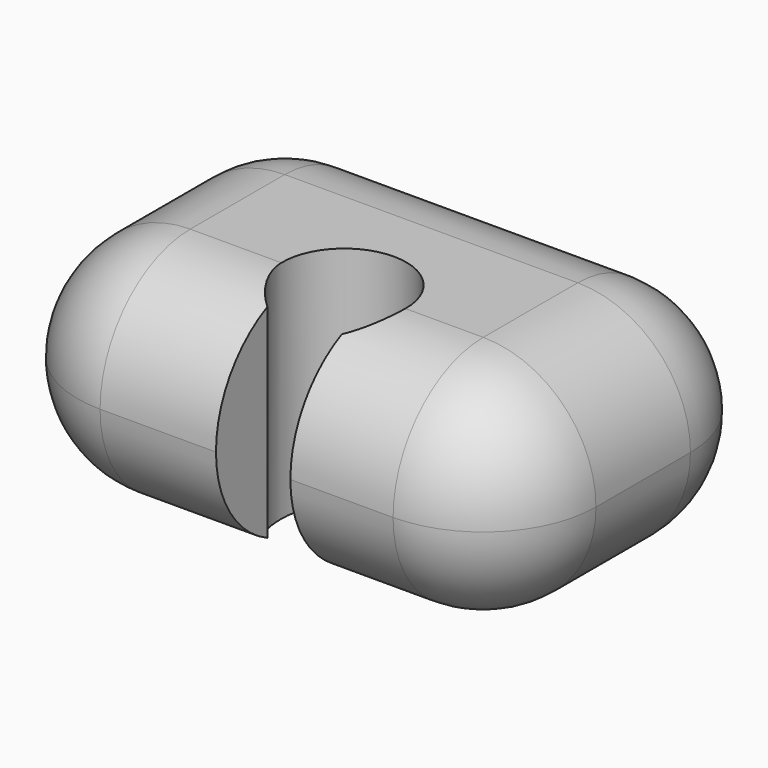
from build123d import *

# Parameters (mm, degrees)
F1_DEPTH = 10
F2_R     = 4.99999
F3_R     = 4.99999


# Not quite as in the source:
# - a fillet or chamfer is up to 0.001 mm smaller than in the source, because OpenCascade refuses the exact size


with BuildPart() as f1:
    # F0 (on Top) → F1 (new body)
    with BuildSketch(Plane.XY):
        with BuildLine():
            Line((-11.7916028897, 0), (-1.65, 0))
            Line((-1.65, 0), (-1.65, 2.85))
            ThreePointArc((-1.65, 2.85), (-1.2298373876, 7.5096747752), (2.75, 5.05))
            ThreePointArc((2.75, 5.05), (2.4596747752, 3.8201626124), (1.65, 2.85))
            Line((1.65, 2.85), (1.65, 0))
            Line((1.65, 0), (11.2060164511, 0))
            Line((11.2060164511, 0), (11.2060164511, 15.24))
            Line((11.2060164511, 15.24), (-11.7916028897, 15.24))
            Line((-11.7916028897, 15.24), (-11.7916028897, 0))
        make_face()
    extrude(amount=F1_DEPTH)

    # F2 (radius 5 in the source; OpenCascade refuses exactly that, so slightly less here)
    f2_edges = [f1.edges().sort_by_distance(p)[0] for p in [
        (11.206016, 7.62, 10),
        (11.206016, 7.62, 0),
        (-11.791603, 7.62, 0),
        (-11.791603, 7.62, 10),
    ]]
    fillet(f2_edges, radius=F2_R)

    # F3 (radius 5 in the source; OpenCascade refuses exactly that, so slightly less here)
    f3_edges = [f1.edges().sort_by_distance(p)[0] for p in [
        (-0.292793, 15.24, 10),
        (-10.32714, 0, 1.464463),
        (9.741553, 0, 1.464463),
    ]]
    fillet(f3_edges, radius=F3_R)


solid = f1.part
